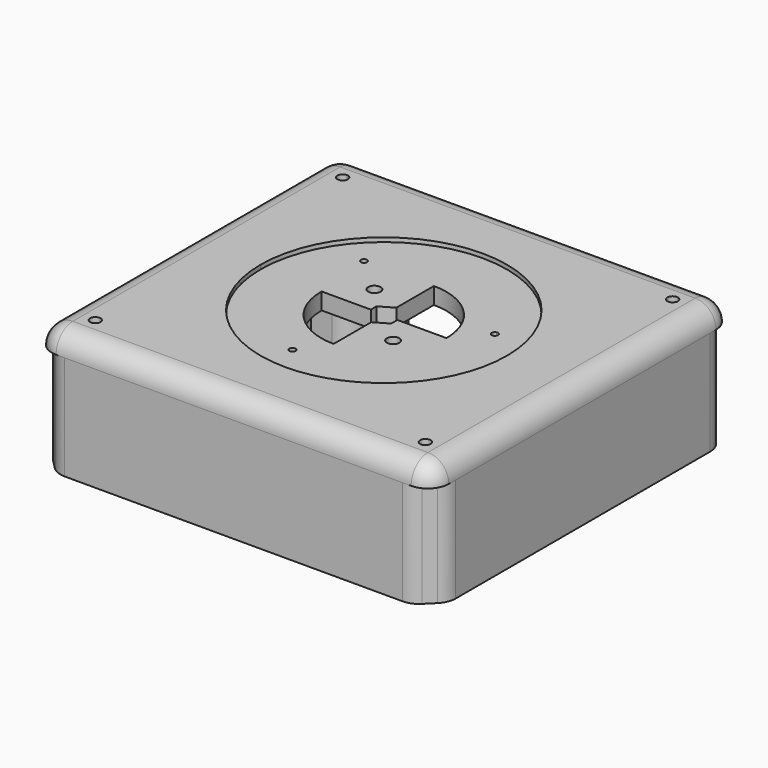
from build123d import *

# Parameters (mm, degrees)
F0_R     = 1.25
F0_R_2   = 1.5
F0_R_3   = 0.75
F1_DEPTH = 5
F2_DEPTH = 1
F3_R     = 4.99999
F4_W     = 10
F4_H     = 25
F4_R     = 1.25
F4_H_2   = 50
F5_DEPTH = 25
F6_R     = 5


# Not quite as in the source:
# - a fillet or chamfer is up to 0.001 mm smaller than in the source, because OpenCascade refuses the exact size
# - a feature names something its author has since deleted; it is built from what else it names


with BuildPart() as f1:
    # F0 (on Top) → F1 (new body)
    with BuildSketch(Plane.XY):
        Polygon((-47.5, 45), (-47.5, 0), (-47.5, -45), (0, -45), (47.5, -45), (47.5, 0), (47.5, 45), (0, 45), (-39.5, 45), align=None)
        with Locations((-39.5, -37)):
            Circle(F0_R, mode=Mode.SUBTRACT)
        with Locations((39.5, -37)):
            Circle(F0_R, mode=Mode.SUBTRACT)
        with BuildLine():
            ThreePointArc((-29.415100958, -0.1703659098), (-29.4149779713, -0.0851825998), (-29.4146090124, 0))
            ThreePointArc((-29.4146090124, 0), (-20.7144303421, 20.7494308667), (0.084899042, 29.3296340902))
            ThreePointArc((0.084899042, 29.3296340902), (20.944549087, 20.6892841352), (29.584899042, -0.1703659098))
            ThreePointArc((29.584899042, -0.1703659098), (23.8481068353, -17.6506392307), (8.8689698641, -28.3322213137))
            ThreePointArc((8.8689698641, -28.3322213137), (4.5276046132, -29.3339110854), (0.084899042, -29.6703659098))
            ThreePointArc((0.084899042, -29.6703659098), (-20.774751003, -21.0300159548), (-29.415100958, -0.1703659098))
        make_face(mode=Mode.SUBTRACT)
        with BuildLine():
            ThreePointArc((-38.25, 37), (-40.3838834765, 36.1161165235), (-39.5, 38.25))
            ThreePointArc((-39.5, 38.25), (-38.6161165235, 37.8838834765), (-38.25, 37))
        make_face(mode=Mode.SUBTRACT)
        with Locations((39.5, 37)):
            Circle(F0_R, mode=Mode.SUBTRACT)
        with BuildLine():
            Line((0.084899042, 29.3296340902), (0.084899042, 14.8296340902))
            ThreePointArc((0.084899042, 14.8296340902), (10.6915007598, 10.436235808), (15.084899042, -0.1703659098))
            Line((15.084899042, -0.1703659098), (29.584899042, -0.1703659098))
            ThreePointArc((29.584899042, -0.1703659098), (20.944549087, 20.6892841352), (0.084899042, 29.3296340902))
        make_face()
        Polygon((17.6671119439, 8.3875283412), (20.791260429, 10.5692011497), (24.2427187464, 8.9544456008), (24.5700285789, 5.1580172433), (21.4458800938, 2.9763444347), (17.9944217764, 4.5910999837), align=None, mode=Mode.SUBTRACT)
        with BuildLine():
            Line((29.584899042, -0.1703659098), (15.084899042, -0.1703659098))
            ThreePointArc((15.084899042, -0.1703659098), (10.6915007598, -10.7769676276), (0.084899042, -15.1703659098))
            Line((0.084899042, -15.1703659098), (0.084899042, -22.7929762808))
            Line((0.084899042, -22.7929762808), (0.084899042, -25.415358255))
            Line((0.084899042, -25.415358255), (0.084899042, -29.6703659098))
            ThreePointArc((0.084899042, -29.6703659098), (4.5276046132, -29.3339110854), (8.8689698641, -28.3322213137))
            ThreePointArc((8.8689698641, -28.3322213137), (23.8481068353, -17.6506392307), (29.584899042, -0.1703659098))
        make_face()
        with BuildLine():
            Line((-29.4146090124, 0), (-14.914133442, 0))
            ThreePointArc((-14.914133442, 0), (-10.4612972237, 10.4962991887), (0.084899042, 14.8296340902))
            Line((0.084899042, 14.8296340902), (0.084899042, 29.3296340902))
            ThreePointArc((0.084899042, 29.3296340902), (-20.7144303421, 20.7494308667), (-29.4146090124, 0))
        make_face()
        Polygon((-18.3295369154, 17.5667340919), (-14.7952109651, 17.7024147245), (-12.9105451153, 14.7094389826), (-14.5602052158, 11.5807826081), (-18.0945311661, 11.4451019755), (-19.9791970159, 14.4380777174), align=None, mode=Mode.SUBTRACT)
        with BuildLine():
            ThreePointArc((-2.9651468575, -14.8569999697), (-11.5501920297, -9.6373958428), (-14.915100958, -0.1703659098))
            Line((-14.915100958, -0.1703659098), (-29.415100958, -0.1703659098))
            ThreePointArc((-29.415100958, -0.1703659098), (-20.774751003, -21.0300159548), (0.084899042, -29.6703659098))
            Line((0.084899042, -29.6703659098), (0.084899042, -25.415358255))
            Line((0.084899042, -25.415358255), (0.084899042, -22.7929762808))
            Line((0.084899042, -22.7929762808), (-1.0164592122, -22.5642517676))
            Line((-1.0164592122, -22.5642517676), (-2.5137461813, -25.1576288716))
            Line((-2.5137461813, -25.1576288716), (-6.324257958, -25.1576288716))
            Line((-6.324257958, -25.1576288716), (-8.2295138463, -21.8576288716))
            Line((-8.2295138463, -21.8576288716), (-6.324257958, -18.5576288716))
            Line((-6.324257958, -18.5576288716), (-3.7336747559, -18.5576288716))
            Line((-3.7336747559, -18.5576288716), (-2.9651468575, -14.8569999697))
        make_face()
        with BuildLine():
            Line((15.084899042, -0.1703659098), (6.084899042, -0.1703659098))
            ThreePointArc((6.084899042, -0.1703659098), (4.3275397292, -4.4130065969), (0.084899042, -6.1703659098))
            Line((0.084899042, -6.1703659098), (0.084899042, -15.1703659098))
            ThreePointArc((0.084899042, -15.1703659098), (10.6915007598, -10.7769676276), (15.084899042, -0.1703659098))
        make_face()
        with Locations((7.9206817116, -7.159679893)):
            Circle(F0_R_2, mode=Mode.SUBTRACT)
        with BuildLine():
            Line((-14.914133442, 0), (-5.9126817583, 0))
            ThreePointArc((-5.9126817583, 0), (-4.0970744479, 4.1320866151), (0.084899042, 5.8296340902))
            Line((0.084899042, 5.8296340902), (0.084899042, 14.8296340902))
            ThreePointArc((0.084899042, 14.8296340902), (-10.4612972237, 10.4962991887), (-14.914133442, 0))
        make_face()
        with Locations((-7.7508836275, 6.8189480734)):
            Circle(F0_R_2, mode=Mode.SUBTRACT)
        Polygon((24.2427187464, 8.9544456008), (20.791260429, 10.5692011497), (17.6671119439, 8.3875283412), (17.9944217764, 4.5910999837), (21.4458800938, 2.9763444347), (24.5700285789, 5.1580172433), align=None)
        with Locations((21.1185702614, 6.7727727922)):
            Circle(F0_R_3, mode=Mode.SUBTRACT)
        Polygon((-12.9105451153, 14.7094389826), (-14.7952109651, 17.7024147245), (-18.3295369154, 17.5667340919), (-19.9791970159, 14.4380777174), (-18.0945311661, 11.4451019755), (-14.5602052158, 11.5807826081), align=None)
        with Locations((-16.4448710656, 14.57375835)):
            Circle(F0_R_3, mode=Mode.SUBTRACT)
        with BuildLine():
            Line((-4.2664997747, -21.1232971686), (-3.7336747559, -18.5576288716))
            Line((-3.7336747559, -18.5576288716), (-6.324257958, -18.5576288716))
            Line((-6.324257958, -18.5576288716), (-8.2295138463, -21.8576288716))
            Line((-8.2295138463, -21.8576288716), (-6.324257958, -25.1576288716))
            Line((-6.324257958, -25.1576288716), (-2.5137461813, -25.1576288716))
            Line((-2.5137461813, -25.1576288716), (-1.0164592122, -22.5642517676))
            Line((-1.0164592122, -22.5642517676), (-3.6846703667, -22.0101311666))
            ThreePointArc((-3.6846703667, -22.0101311666), (-5.0460884034, -22.2690443915), (-4.2664997747, -21.1232971686))
        make_face()
        with BuildLine():
            ThreePointArc((0.084899042, -6.1703659098), (4.3275397292, -4.4130065969), (6.084899042, -0.1703659098))
            Line((6.084899042, -0.1703659098), (3.334899042, -0.1703659098))
            Line((3.334899042, -0.1703659098), (3.334899042, -2.0467542847))
            Line((3.334899042, -2.0467542847), (0.084899042, -3.9231426595))
            Line((0.084899042, -3.9231426595), (0.084899042, -6.1703659098))
        make_face()
        with BuildLine():
            Line((-5.9126817583, 0), (-3.165100958, 0))
            Line((-3.165100958, 0), (-3.165100958, 1.7060224651))
            Line((-3.165100958, 1.7060224651), (0.084899042, 3.5824108399))
            Line((0.084899042, 3.5824108399), (0.084899042, 5.8296340902))
            ThreePointArc((0.084899042, 5.8296340902), (-4.0970744479, 4.1320866151), (-5.9126817583, 0))
        make_face()
        with BuildLine():
            ThreePointArc((0.084899042, -15.1703659098), (-1.4481516911, -15.0918187697), (-2.9651468575, -14.8569999697))
            Line((-2.9651468575, -14.8569999697), (-3.7336747559, -18.5576288716))
            Line((-3.7336747559, -18.5576288716), (-2.5137461813, -18.5576288716))
            Line((-2.5137461813, -18.5576288716), (-0.608490293, -21.8576288716))
            Line((-0.608490293, -21.8576288716), (-1.0164592122, -22.5642517676))
            Line((-1.0164592122, -22.5642517676), (0.084899042, -22.7929762808))
            Line((0.084899042, -22.7929762808), (0.084899042, -15.1703659098))
        make_face()
        with BuildLine():
            Line((-2.5137461813, -18.5576288716), (-3.7336747559, -18.5576288716))
            Line((-3.7336747559, -18.5576288716), (-4.2664997747, -21.1232971686))
            ThreePointArc((-4.2664997747, -21.1232971686), (-3.8372475161, -21.384277375), (-3.6690020697, -21.8576288716))
            ThreePointArc((-3.6690020697, -21.8576288716), (-3.6729294267, -21.9342814083), (-3.6846703667, -22.0101311666))
            Line((-3.6846703667, -22.0101311666), (-1.0164592122, -22.5642517676))
            Line((-1.0164592122, -22.5642517676), (-0.608490293, -21.8576288716))
            Line((-0.608490293, -21.8576288716), (-2.5137461813, -18.5576288716))
        make_face()
        with BuildLine():
            ThreePointArc((-14.915100958, -0.1703659098), (-14.914859077, -0.0851815813), (-14.914133442, 0))
            Line((-14.914133442, 0), (-29.4146090124, 0))
            ThreePointArc((-29.4146090124, 0), (-29.4149779713, -0.0851825998), (-29.415100958, -0.1703659098))
            Line((-29.415100958, -0.1703659098), (-14.915100958, -0.1703659098))
        make_face()
    extrude(amount=-F1_DEPTH)

    # F0 (on Top) → F2 (cut)
    with BuildSketch(Plane.XY):
        with BuildLine():
            Line((-5.9126817583, 0), (-3.165100958, 0))
            Line((-3.165100958, 0), (-3.165100958, 1.7060224651))
            Line((-3.165100958, 1.7060224651), (0.084899042, 3.5824108399))
            Line((0.084899042, 3.5824108399), (0.084899042, 5.8296340902))
            ThreePointArc((0.084899042, 5.8296340902), (-4.0970744479, 4.1320866151), (-5.9126817583, 0))
        make_face()
        with BuildLine():
            Line((-14.914133442, 0), (-5.9126817583, 0))
            ThreePointArc((-5.9126817583, 0), (-4.0970744479, 4.1320866151), (0.084899042, 5.8296340902))
            Line((0.084899042, 5.8296340902), (0.084899042, 14.8296340902))
            ThreePointArc((0.084899042, 14.8296340902), (-10.4612972237, 10.4962991887), (-14.914133442, 0))
        make_face()
        with Locations((-7.7508836275, 6.8189480734)):
            Circle(F0_R_2, mode=Mode.SUBTRACT)
        with BuildLine():
            ThreePointArc((-14.915100958, -0.1703659098), (-14.914859077, -0.0851815813), (-14.914133442, 0))
            Line((-14.914133442, 0), (-29.4146090124, 0))
            ThreePointArc((-29.4146090124, 0), (-29.4149779713, -0.0851825998), (-29.415100958, -0.1703659098))
            Line((-29.415100958, -0.1703659098), (-14.915100958, -0.1703659098))
        make_face()
        with BuildLine():
            Line((-29.4146090124, 0), (-14.914133442, 0))
            ThreePointArc((-14.914133442, 0), (-10.4612972237, 10.4962991887), (0.084899042, 14.8296340902))
            Line((0.084899042, 14.8296340902), (0.084899042, 29.3296340902))
            ThreePointArc((0.084899042, 29.3296340902), (-20.7144303421, 20.7494308667), (-29.4146090124, 0))
        make_face()
        Polygon((-18.3295369154, 17.5667340919), (-14.7952109651, 17.7024147245), (-12.9105451153, 14.7094389826), (-14.5602052158, 11.5807826081), (-18.0945311661, 11.4451019755), (-19.9791970159, 14.4380777174), align=None, mode=Mode.SUBTRACT)
        with BuildLine():
            Line((0.084899042, 29.3296340902), (0.084899042, 14.8296340902))
            ThreePointArc((0.084899042, 14.8296340902), (10.6915007598, 10.436235808), (15.084899042, -0.1703659098))
            Line((15.084899042, -0.1703659098), (29.584899042, -0.1703659098))
            ThreePointArc((29.584899042, -0.1703659098), (20.944549087, 20.6892841352), (0.084899042, 29.3296340902))
        make_face()
        Polygon((17.6671119439, 8.3875283412), (20.791260429, 10.5692011497), (24.2427187464, 8.9544456008), (24.5700285789, 5.1580172433), (21.4458800938, 2.9763444347), (17.9944217764, 4.5910999837), align=None, mode=Mode.SUBTRACT)
        with BuildLine():
            ThreePointArc((-2.9651468575, -14.8569999697), (-11.5501920297, -9.6373958428), (-14.915100958, -0.1703659098))
            Line((-14.915100958, -0.1703659098), (-29.415100958, -0.1703659098))
            ThreePointArc((-29.415100958, -0.1703659098), (-20.774751003, -21.0300159548), (0.084899042, -29.6703659098))
            Line((0.084899042, -29.6703659098), (0.084899042, -25.415358255))
            Line((0.084899042, -25.415358255), (0.084899042, -22.7929762808))
            Line((0.084899042, -22.7929762808), (-1.0164592122, -22.5642517676))
            Line((-1.0164592122, -22.5642517676), (-2.5137461813, -25.1576288716))
            Line((-2.5137461813, -25.1576288716), (-6.324257958, -25.1576288716))
            Line((-6.324257958, -25.1576288716), (-8.2295138463, -21.8576288716))
            Line((-8.2295138463, -21.8576288716), (-6.324257958, -18.5576288716))
            Line((-6.324257958, -18.5576288716), (-3.7336747559, -18.5576288716))
            Line((-3.7336747559, -18.5576288716), (-2.9651468575, -14.8569999697))
        make_face()
        with BuildLine():
            ThreePointArc((0.084899042, -6.1703659098), (4.3275397292, -4.4130065969), (6.084899042, -0.1703659098))
            Line((6.084899042, -0.1703659098), (3.334899042, -0.1703659098))
            Line((3.334899042, -0.1703659098), (3.334899042, -2.0467542847))
            Line((3.334899042, -2.0467542847), (0.084899042, -3.9231426595))
            Line((0.084899042, -3.9231426595), (0.084899042, -6.1703659098))
        make_face()
        with BuildLine():
            Line((15.084899042, -0.1703659098), (6.084899042, -0.1703659098))
            ThreePointArc((6.084899042, -0.1703659098), (4.3275397292, -4.4130065969), (0.084899042, -6.1703659098))
            Line((0.084899042, -6.1703659098), (0.084899042, -15.1703659098))
            ThreePointArc((0.084899042, -15.1703659098), (10.6915007598, -10.7769676276), (15.084899042, -0.1703659098))
        make_face()
        with Locations((7.9206817116, -7.159679893)):
            Circle(F0_R_2, mode=Mode.SUBTRACT)
        with BuildLine():
            Line((29.584899042, -0.1703659098), (15.084899042, -0.1703659098))
            ThreePointArc((15.084899042, -0.1703659098), (10.6915007598, -10.7769676276), (0.084899042, -15.1703659098))
            Line((0.084899042, -15.1703659098), (0.084899042, -22.7929762808))
            Line((0.084899042, -22.7929762808), (0.084899042, -25.415358255))
            Line((0.084899042, -25.415358255), (0.084899042, -29.6703659098))
            ThreePointArc((0.084899042, -29.6703659098), (4.5276046132, -29.3339110854), (8.8689698641, -28.3322213137))
            ThreePointArc((8.8689698641, -28.3322213137), (23.8481068353, -17.6506392307), (29.584899042, -0.1703659098))
        make_face()
        with BuildLine():
            ThreePointArc((0.084899042, -15.1703659098), (-1.4481516911, -15.0918187697), (-2.9651468575, -14.8569999697))
            Line((-2.9651468575, -14.8569999697), (-3.7336747559, -18.5576288716))
            Line((-3.7336747559, -18.5576288716), (-2.5137461813, -18.5576288716))
            Line((-2.5137461813, -18.5576288716), (-0.608490293, -21.8576288716))
            Line((-0.608490293, -21.8576288716), (-1.0164592122, -22.5642517676))
            Line((-1.0164592122, -22.5642517676), (0.084899042, -22.7929762808))
            Line((0.084899042, -22.7929762808), (0.084899042, -15.1703659098))
        make_face()
        with BuildLine():
            Line((-2.5137461813, -18.5576288716), (-3.7336747559, -18.5576288716))
            Line((-3.7336747559, -18.5576288716), (-4.2664997747, -21.1232971686))
            ThreePointArc((-4.2664997747, -21.1232971686), (-3.8372475161, -21.384277375), (-3.6690020697, -21.8576288716))
            ThreePointArc((-3.6690020697, -21.8576288716), (-3.6729294267, -21.9342814083), (-3.6846703667, -22.0101311666))
            Line((-3.6846703667, -22.0101311666), (-1.0164592122, -22.5642517676))
            Line((-1.0164592122, -22.5642517676), (-0.608490293, -21.8576288716))
            Line((-0.608490293, -21.8576288716), (-2.5137461813, -18.5576288716))
        make_face()
        with BuildLine():
            Line((-4.2664997747, -21.1232971686), (-3.7336747559, -18.5576288716))
            Line((-3.7336747559, -18.5576288716), (-6.324257958, -18.5576288716))
            Line((-6.324257958, -18.5576288716), (-8.2295138463, -21.8576288716))
            Line((-8.2295138463, -21.8576288716), (-6.324257958, -25.1576288716))
            Line((-6.324257958, -25.1576288716), (-2.5137461813, -25.1576288716))
            Line((-2.5137461813, -25.1576288716), (-1.0164592122, -22.5642517676))
            Line((-1.0164592122, -22.5642517676), (-3.6846703667, -22.0101311666))
            ThreePointArc((-3.6846703667, -22.0101311666), (-5.0460884034, -22.2690443915), (-4.2664997747, -21.1232971686))
        make_face()
        Polygon((-12.9105451153, 14.7094389826), (-14.7952109651, 17.7024147245), (-18.3295369154, 17.5667340919), (-19.9791970159, 14.4380777174), (-18.0945311661, 11.4451019755), (-14.5602052158, 11.5807826081), align=None)
        with Locations((-16.4448710656, 14.57375835)):
            Circle(F0_R_3, mode=Mode.SUBTRACT)
        Polygon((24.2427187464, 8.9544456008), (20.791260429, 10.5692011497), (17.6671119439, 8.3875283412), (17.9944217764, 4.5910999837), (21.4458800938, 2.9763444347), (24.5700285789, 5.1580172433), align=None)
        with Locations((21.1185702614, 6.7727727922)):
            Circle(F0_R_3, mode=Mode.SUBTRACT)
    extrude(amount=-F2_DEPTH, mode=Mode.SUBTRACT)

    # F3 (radius 5 in the source; OpenCascade refuses exactly that, so slightly less here)
    f3_edges = [f1.edges().sort_by_distance(p)[0] for p in [
        (-47.5, 0, 0),
        (0, 45, 0),
        (0, -45, 0),
        (47.5, 0, 0),
        (47.5, -45, -2.5),
        (-47.5, -45, -2.5),
        (-47.5, 45, -2.5),
        (47.5, 45, -2.5),
    ]]
    fillet(f3_edges, radius=F3_R)


with BuildPart() as f5:
    # F4 (on face) → F5 (new body)
    with BuildSketch(Plane(origin=(0, 0, -5), x_dir=(1, 0, 0), z_dir=(0, 0, -1))):
        Polygon((-27.5, 45), (-39.5, 45), (-42.5, 45), (-47.5, 40), (-47.5, 25), (-37.5, 25), (-27.5, 25), (-27.5, 35), align=None)
        with BuildLine():
            ThreePointArc((-38.25, 37), (-40.3838834765, 36.1161165235), (-39.5, 38.25))
            ThreePointArc((-39.5, 38.25), (-38.6161165235, 37.8838834765), (-38.25, 37))
        make_face(mode=Mode.SUBTRACT)
        Polygon((0, 45), (-27.5, 45), (-27.5, 35), (27.5, 35), (27.5, 45), align=None)
        with Locations((-42.5, 12.5)):
            Rectangle(F4_W, F4_H)
        Polygon((42.5, 45), (27.5, 45), (27.5, 35), (27.5, 25), (37.5, 25), (47.5, 25), (47.5, 40), align=None)
        with Locations((39.5, 37)):
            Circle(F4_R, mode=Mode.SUBTRACT)
        with Locations((-42.5, -12.5)):
            Rectangle(F4_W, F4_H)
        Polygon((-37.5, -25), (-47.5, -25), (-47.5, -40), (-42.5, -45), (-27.5, -44.9826236297), (-27.5, -35), (-27.5, -25), align=None)
        with Locations((-39.5, -37)):
            Circle(F4_R, mode=Mode.SUBTRACT)
        with Locations((42.5, 0)):
            Rectangle(F4_W, F4_H_2)
        Polygon((47.5, -25), (37.5, -25), (27.5, -25), (27.5, -35), (27.5, -44.9189102719), (43.4930970818, -44.9003834734), (47.5, -40), align=None)
        with Locations((39.5, -37)):
            Circle(F4_R, mode=Mode.SUBTRACT)
    extrude(amount=F5_DEPTH)

    # F6
    f6_edges = [f5.edges().sort_by_distance(p)[0] for p in [
        (-42.5, -45, -17.5),
        (42.5, -45, -17.5),
        (47.5, -40, -17.5),
        (47.5, 40, -17.5),
        (43.493097, 44.900383, -17.5),
        (-42.5, 45, -17.5),
        (-47.5, 40, -17.5),
        (-27.5, 44.982624, -17.5),
        (27.5, -25, -17.5),
        (-27.5, -25, -17.5),
        (-27.5, 25, -17.5),
        (27.5, 25, -17.5),
        (-47.5, -40, -17.5),
        (27.5, 44.91891, -17.5),
    ]]
    fillet(f6_edges, radius=F6_R)


solid = Compound([f1.part, f5.part])
